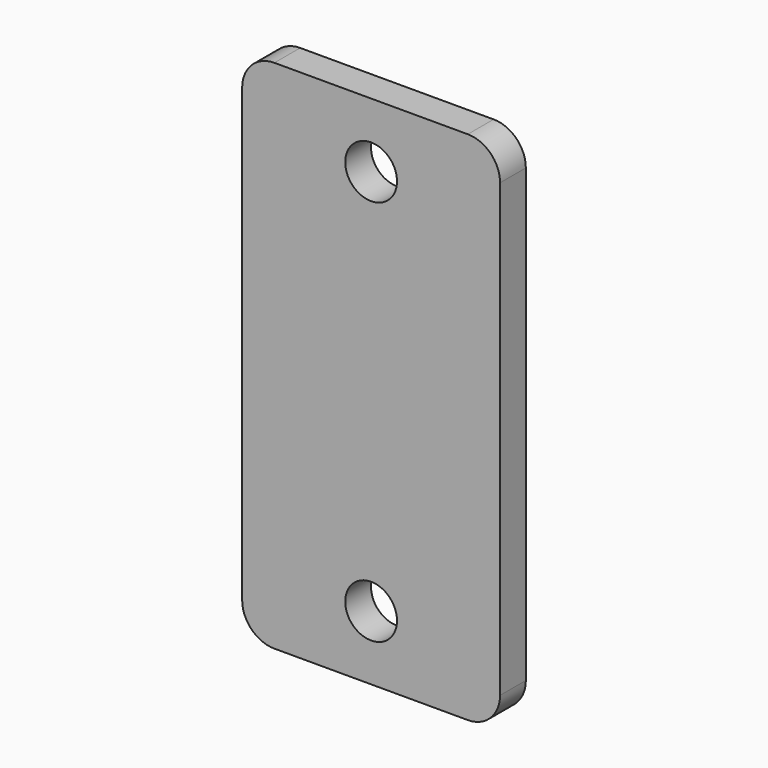
from build123d import *

# Parameters (mm, degrees)
F1_W     = 25.4
F1_H     = 50.8
F1_R     = 2.55
F2_DEPTH = 3.175
F3_R     = 3.175


# Not quite as in the source:
# - a variable given as a bare number and used for a length is read in inches; the dataset says mm whatever the document's units were


with BuildPart() as f2:
    # F1 (on Front) → F2 (new body)
    with BuildSketch(Plane.XZ):
        Rectangle(F1_W, F1_H)
        with Locations((0, -19.05)):
            Circle(F1_R, mode=Mode.SUBTRACT)
        with Locations((0, 19.05)):
            Circle(F1_R, mode=Mode.SUBTRACT)
    extrude(amount=F2_DEPTH)

    # F3
    f3_edges = [f2.edges().sort_by_distance(p)[0] for p in [
        (-12.7, -1.5875, 25.4),
        (12.7, -1.5875, 25.4),
        (12.7, -1.5875, -25.4),
        (-12.7, -1.5875, -25.4),
    ]]
    fillet(f3_edges, radius=F3_R)


solid = f2.part
